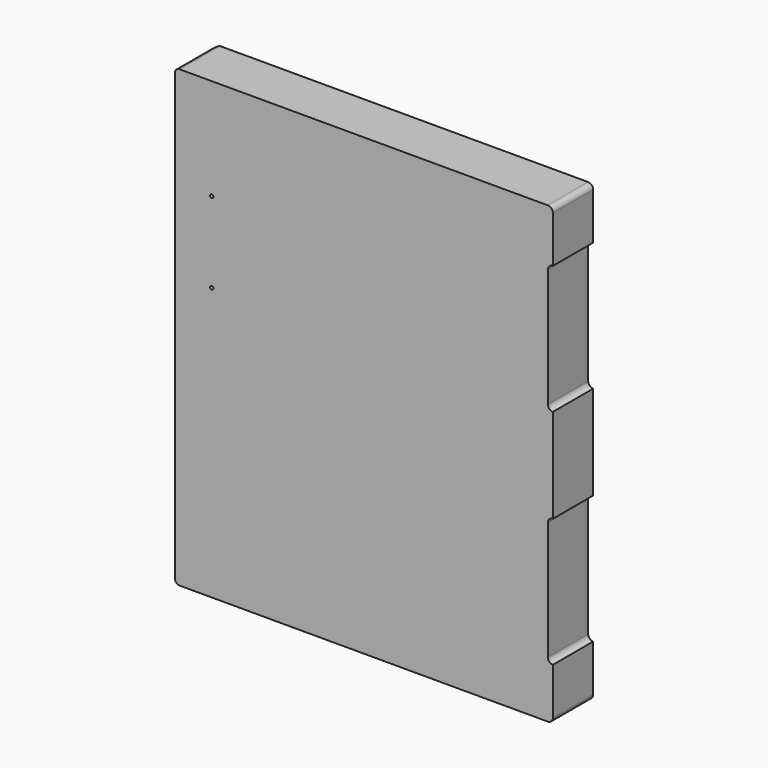
from build123d import *

# Parameters (mm, degrees)
F0_W          = 225
F0_H          = 270.5
F1_DEPTH      = 30
F2_R          = 3
F3_W          = 30
F3_H          = 76.5
F4_DEPTH      = 3
F5_R          = 2.99999
F6_W          = 21
F6_H          = 238
F7_DEPTH      = 3
F8_R          = 2.99999
F9_W          = 21
F9_H          = 145
F10_DEPTH     = 61
F11_R         = 3
F12_T1_DEPTH  = 28.6800979278
F12_T3_DEPTH  = 28.6800979278
F12_T8_DEPTH  = 15.4301079278
F12_T13_DEPTH = 15.4301079278
F13_W         = 61
F13_H         = 13
F14_DEPTH     = 5
F15_R         = 3
F16_R         = 1
F17_DEPTH     = 25


# Not quite as in the source:
# - a fillet or chamfer that OpenCascade refuses, or shapes differently, is made with other operations: its cross-section is extruded or revolved along the edge and cut away or added
# - a fillet or chamfer is up to 0.001 mm smaller than in the source, because OpenCascade refuses the exact size


with BuildPart() as f1:
    # F0 (on Front) → F1 (new body)
    with BuildSketch(Plane.XZ):
        Rectangle(F0_W, F0_H)
    extrude(amount=F1_DEPTH)

    # F2
    f2_edges = [f1.edges().sort_by_distance(p)[0] for p in [
        (112.5, -15, 135.25),
        (112.5, -15, -135.25),
        (-112.5, -15, 135.25),
        (-112.5, -15, -135.25),
    ]]
    fillet(f2_edges, radius=F2_R)

    # F3 (on face) → F4 (cut)
    with BuildSketch(Plane.YZ.offset(112.5)):
        with Locations((-15, 66.25)):
            Rectangle(F3_W, F3_H)
        with Locations((-15, -66.25)):
            Rectangle(F3_W, F3_H)
    extrude(amount=-F4_DEPTH, mode=Mode.SUBTRACT)

    # F5 (radius 3 in the source; OpenCascade refuses exactly that, so slightly less here)
    f5_edges = [f1.edges().sort_by_distance(p)[0] for p in [
        (109.5, -15, 28),
        (109.5, -15, -104.5),
        (109.5, -15, -28),
        (109.5, -15, 104.5),
    ]]
    fillet(f5_edges, radius=F5_R)

    # F6 (on face) → F7 (cut)
    with BuildSketch(Plane(origin=(-112.5, 0, 0), x_dir=(0, -1, 0), z_dir=(-1, 0, 0))):
        with Locations((10.5, 0)):
            Rectangle(F6_W, F6_H)
    extrude(amount=-F7_DEPTH, mode=Mode.SUBTRACT)

    # F8 (radius 3 in the source; OpenCascade refuses exactly that, so slightly less here)
    f8_edges = [f1.edges().sort_by_distance(p)[0] for p in [
        (-109.5, -10.5, -119),
        (-109.5, -10.5, 119),
    ]]
    fillet(f8_edges, radius=F8_R)

    # F9 (on face) → F10 (cut)
    with BuildSketch(Plane(origin=(-109.5, 0, 0), x_dir=(0, -1, 0), z_dir=(-1, 0, 0))):
        with Locations((10.5, 0)):
            Rectangle(F9_W, F9_H)
    extrude(amount=-F10_DEPTH, mode=Mode.SUBTRACT)

    # F11
    f11_edges = [f1.edges().sort_by_distance(p)[0] for p in [
        (-48.5, -10.5, -72.5),
        (-48.5, -10.5, 72.5),
    ]]
    fillet(f11_edges, radius=F11_R)

    # F12: chamfer of 3 on 6 edges, made by hand

    # F12_s2 → F12_t1 (cut)
    with BuildSketch(Plane.XY.offset(-139.9650489639)):
        Polygon((-109.5, 0), (-112.5, -3), (-112.5, 0), align=None)
    extrude(amount=F12_T1_DEPTH, mode=Mode.SUBTRACT)

    # F12_s4 → F12_t3 (cut)
    with BuildSketch(Plane.XY.offset(111.2849510361)):
        Polygon((-109.5, 0), (-112.5, -3), (-112.5, 0), align=None)
    extrude(amount=F12_T3_DEPTH, mode=Mode.SUBTRACT)


with BuildPart() as f12_tool6:
    # F12_s7 → F12_t8 (new body)
    with BuildSketch(Plane.YZ.offset(-120.2150489639)):
        Polygon((0, -122), (-3, -119), (0, -119), align=None)
    extrude(amount=F12_T8_DEPTH)

    split(bisect_by=Plane(origin=(-54.75, 54.75, 0), x_dir=(0, 0, 1), z_dir=(-0.7071067812, 0.7071067812, 0)), keep=Keep.TOP)


with BuildPart() as f1_1:
    add(f1.part)

    # F12_t5: cut F12_tool6
    add(f12_tool6.part, mode=Mode.SUBTRACT)


with BuildPart() as f12_tool11:
    # F12_s12 → F12_t13 (new body)
    with BuildSketch(Plane.YZ.offset(-120.2150489639)):
        Polygon((0, 122), (-3, 119), (0, 119), align=None)
    extrude(amount=F12_T13_DEPTH)

    split(bisect_by=Plane(origin=(-54.75, 54.75, 0), x_dir=(0, 0, 1), z_dir=(-0.7071067812, 0.7071067812, 0)), keep=Keep.TOP)


with BuildPart() as f1_2:
    add(f1_1.part)

    # F12_t10: cut F12_tool11
    add(f12_tool11.part, mode=Mode.SUBTRACT)

    # F13 (on face) → F14 (cut)
    with BuildSketch(Plane(origin=(0, 0, 0), x_dir=(-1, 0, 0), z_dir=(0, 1, 0))):
        with Locations((79, 76)):
            Rectangle(F13_W, F13_H)
    extrude(amount=-F14_DEPTH, mode=Mode.SUBTRACT)

    # F15
    f15_edges = [f1_2.edges().sort_by_distance(p)[0] for p in [
        (-48.5, -2.5, 82.5),
    ]]
    fillet(f15_edges, radius=F15_R)

    # F16 (on face) → F17 (cut)
    with BuildSketch(Plane.XZ.offset(30)):
        with Locations((-90.5, 75)):
            Circle(F16_R)
        with Locations((-90.5, 27)):
            Circle(F16_R)
    extrude(amount=-F17_DEPTH, mode=Mode.SUBTRACT)


solid = f1_2.part
